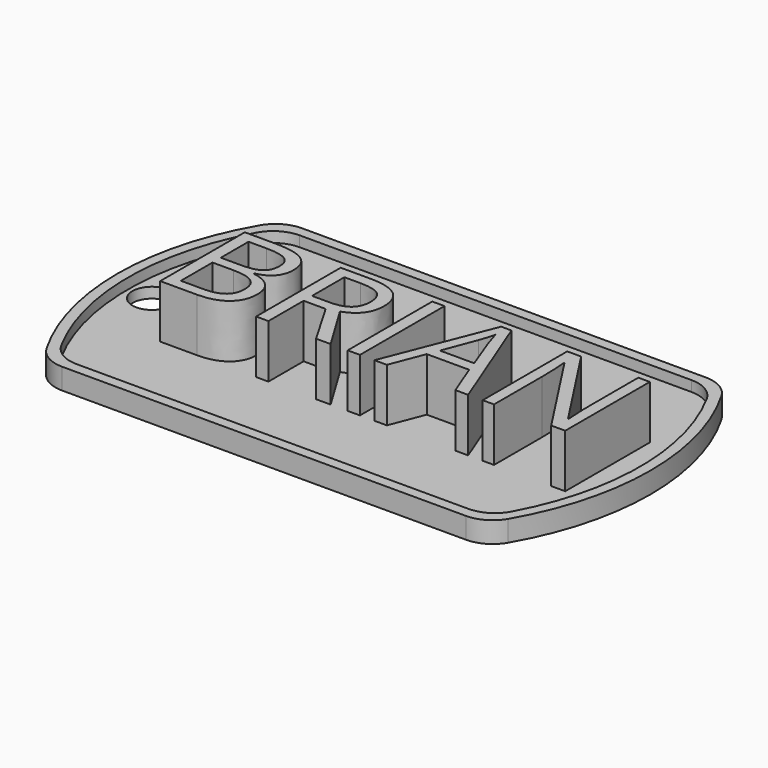
from build123d import *

# Parameters (mm, degrees)
F0_R         = 1.8739594118
F1_DEPTH     = 1
F3_DEPTH     = 1
F4_TEXT_SIZE = 14.1111111111
F5_DEPTH     = 5.08


# Not quite as in the source:
# - Text() gives the source's letters only with a copy of the font that has no kerning and outlines rounded to 1/6400 em; it was checked with that copy


with BuildPart() as f1:
    # F0 (on Top) → F1 (new body)
    with BuildSketch(Plane.XY):
        with BuildLine():
            ThreePointArc((-19.2474145991, 14.2875), (-20.8349145991, 13.862130657), (-21.9970452561, 12.7))
            ThreePointArc((-21.9970452561, 12.7), (-25.4, 0), (-21.9970452561, -12.7))
            ThreePointArc((-21.9970452561, -12.7), (-20.8349145991, -13.862130657), (-19.2474145991, -14.2875))
            Line((-19.2474145991, -14.2875), (19.2474145991, -14.2875))
            ThreePointArc((19.2474145991, -14.2875), (20.8349145991, -13.862130657), (21.9970452561, -12.7))
            ThreePointArc((21.9970452561, -12.7), (25.4, 0), (21.9970452561, 12.7))
            ThreePointArc((21.9970452561, 12.7), (20.8349145991, 13.862130657), (19.2474145991, 14.2875))
            Line((19.2474145991, 14.2875), (-19.2474145991, 14.2875))
        make_face()
        with Locations((-22.0978986472, 0)):
            Circle(F0_R, mode=Mode.SUBTRACT)
    extrude(amount=F1_DEPTH)

    # F2 (on face) → F3 (join)
    with BuildSketch(Plane.XY.offset(1)):
        with BuildLine():
            Line((19.2474145991, 14.2875), (-19.2474145991, 14.2875))
            ThreePointArc((-19.2474145991, 14.2875), (-20.8349145991, 13.862130657), (-21.9970452561, 12.7))
            ThreePointArc((-21.9970452561, 12.7), (-25.4, 0), (-21.9970452561, -12.7))
            ThreePointArc((-21.9970452561, -12.7), (-20.8349145991, -13.862130657), (-19.2474145991, -14.2875))
            Line((-19.2474145991, -14.2875), (19.2474145991, -14.2875))
            ThreePointArc((19.2474145991, -14.2875), (20.8349145991, -13.862130657), (21.9970452561, -12.7))
            ThreePointArc((21.9970452561, -12.7), (25.4, 0), (21.9970452561, 12.7))
            ThreePointArc((21.9970452561, 12.7), (20.8349145991, 13.862130657), (19.2474145991, 14.2875))
        make_face()
        with BuildLine():
            ThreePointArc((-21.4526124879, 11.6252061249), (-20.2856017842, 12.8404540819), (-18.6611352482, 13.2875))
            Line((-18.6611352482, 13.2875), (18.6611352482, 13.2875))
            ThreePointArc((18.6611352482, 13.2875), (20.2856017842, 12.8404540819), (21.4526124879, 11.6252061249))
            ThreePointArc((21.4526124879, 11.6252061249), (24.4, 0), (21.4526124879, -11.6252061249))
            ThreePointArc((21.4526124879, -11.6252061249), (20.2856017842, -12.8404540819), (18.6611352482, -13.2875))
            Line((18.6611352482, -13.2875), (-18.6611352482, -13.2875))
            ThreePointArc((-18.6611352482, -13.2875), (-20.2856017842, -12.8404540819), (-21.4526124879, -11.6252061249))
            ThreePointArc((-21.4526124879, -11.6252061249), (-24.4, 0), (-21.4526124879, 11.6252061249))
        make_face(mode=Mode.SUBTRACT)
    extrude(amount=F3_DEPTH)

    # F4 (on face) → F5 (join)
    with BuildSketch(Plane.XY.offset(1)):
        with Locations((-18.6539742742, -5.0730188003)):
            Text('BRIAN', F4_TEXT_SIZE, font='Open Sans', text_align=(TextAlign.LEFT, TextAlign.BOTTOM))
    extrude(amount=F5_DEPTH)


solid = f1.part
